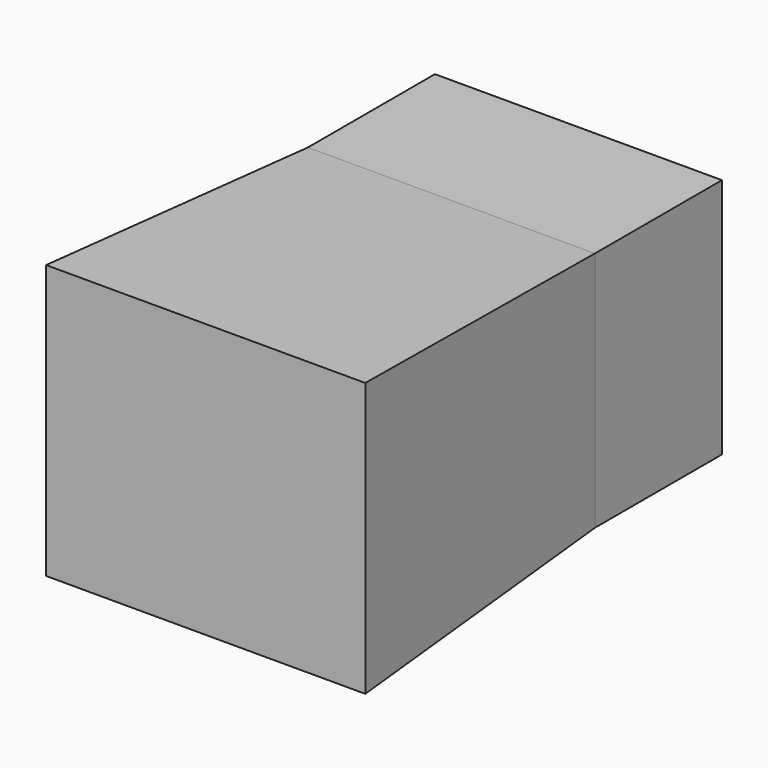
from build123d import *

# Parameters (mm, degrees)
F0_W      = 59.4193041325
F0_H      = 32.8746140003
F1_DEPTH  = 50
F1_FACE_W = 59.4193041325
F1_FACE_H = 50
F2_DEPTH  = 63.5828971863
F2_TAPER  = -3.0006


with BuildPart() as f1:
    # F0 (on Top) → F1 (new body)
    with BuildSketch(Plane.XY):
        with Locations((29.7096520662, -16.4373070002)):
            Rectangle(F0_W, F0_H)
    extrude(amount=F1_DEPTH)

    # F1_face (on face) → F2 (join)
    with BuildSketch(Plane(origin=(29.7096520662, -32.8746140003, 25), x_dir=(1, 0, 0), z_dir=(0, -1, 0))):
        Rectangle(F1_FACE_W, F1_FACE_H)
    extrude(amount=F2_DEPTH, taper=F2_TAPER)


solid = f1.part
